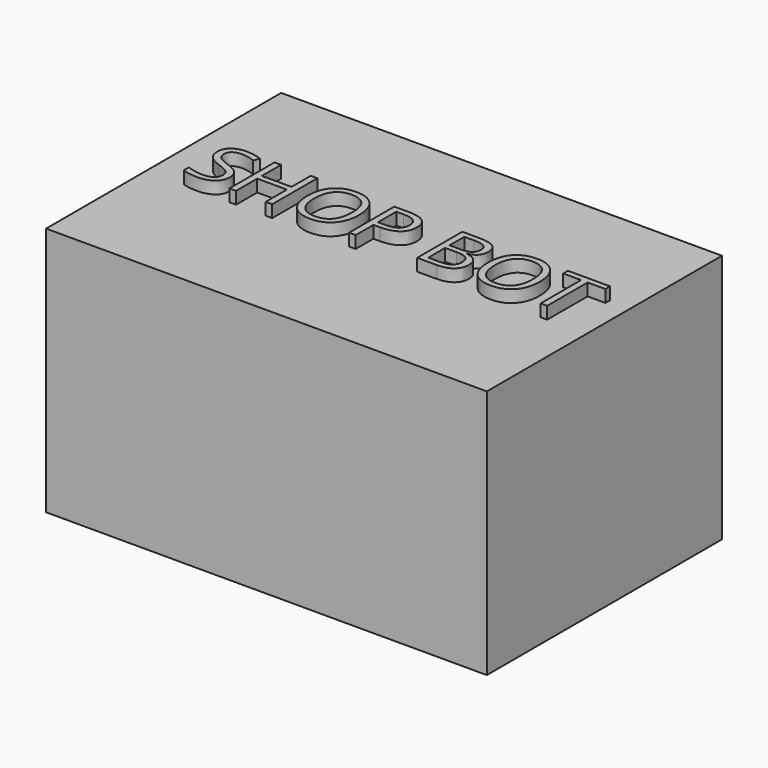
from build123d import *

# Parameters (mm, degrees)
F0_W         = 2743.2
F0_H         = 1828.8
F1_DEPTH     = 1554.48
F2_TEXT_SIZE = 491.3342988477
F3_DEPTH     = 76.2


# Not quite as in the source:
# - Text() gives the source's letters only with a copy of the font that has no kerning and outlines rounded to 1/6400 em; it was checked with that copy


with BuildPart() as f1:
    # F0 (on Top) → F1 (new body)
    with BuildSketch(Plane.XY):
        Rectangle(F0_W, F0_H)
    extrude(amount=F1_DEPTH)

    # F2 (on face) → F3 (join)
    with BuildSketch(Plane.XY.offset(1554.48)):
        with Locations((-1166.1700757178, -142.0587412184)):
            Text('SHOP BOT', F2_TEXT_SIZE, font='Open Sans', text_align=(TextAlign.LEFT, TextAlign.BOTTOM))
    extrude(amount=F3_DEPTH)


solid = f1.part
